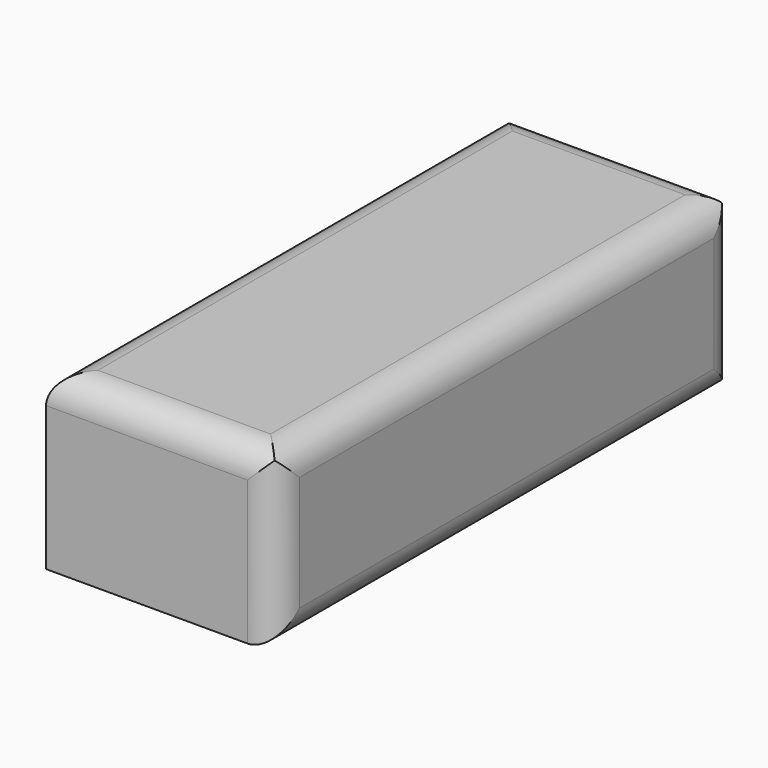
from build123d import *

# Parameters (mm, degrees)
F0_W        = 40
F0_H        = 30
F1_DEPTH    = 50
F2_R        = 5
F3_T1_DEPTH = 50
F3_T3_DEPTH = 125


# Not quite as in the source:
# - a fillet or chamfer that OpenCascade refuses, or shapes differently, is made with other operations: its cross-section is extruded or revolved along the edge and cut away or added


with BuildPart() as f1:
    # F0 (on Front) → F1 (new body, symmetric)
    with BuildSketch(Plane.XZ):
        with Locations((-4.8181314529, -0.4249101039)):
            Rectangle(F0_W, F0_H)
    extrude(amount=F1_DEPTH, both=True)

    # F2
    f2_edges = [f1.edges().sort_by_distance(p)[0] for p in [
        (-4.818131, 50, 14.57509),
        (-24.818131, 0, 14.57509),
        (-4.818131, -50, 14.57509),
        (15.181869, 0, 14.57509),
    ]]
    fillet(f2_edges, radius=F2_R)

    # F3: fillet of radius 5 on 4 edges, made by hand

    # F3_s2 → F3_t1 (cut)
    with BuildSketch(Plane.XY.offset(-27.9249101039)):
        with BuildLine():
            ThreePointArc((10.1818685471, 50), (13.717402453, 48.5355339059), (15.1818685471, 45))
            Line((15.1818685471, 45), (15.1818685471, 50))
            Line((15.1818685471, 50), (10.1818685471, 50))
        make_face()
        with BuildLine():
            ThreePointArc((15.1818685471, -45), (13.717402453, -48.5355339059), (10.1818685471, -50))
            Line((10.1818685471, -50), (15.1818685471, -50))
            Line((15.1818685471, -50), (15.1818685471, -45))
        make_face()
    extrude(amount=F3_T1_DEPTH, mode=Mode.SUBTRACT)

    # F3_s4 → F3_t3 (cut)
    with BuildSketch(Plane.XZ.offset(-62.5)):
        with BuildLine():
            ThreePointArc((15.1818685471, -10.4249101039), (13.717402453, -13.9604440098), (10.1818685471, -15.4249101039))
            Line((10.1818685471, -15.4249101039), (15.1818685471, -15.4249101039))
            Line((15.1818685471, -15.4249101039), (15.1818685471, -10.4249101039))
        make_face()
    extrude(amount=F3_T3_DEPTH, mode=Mode.SUBTRACT)


solid = f1.part
